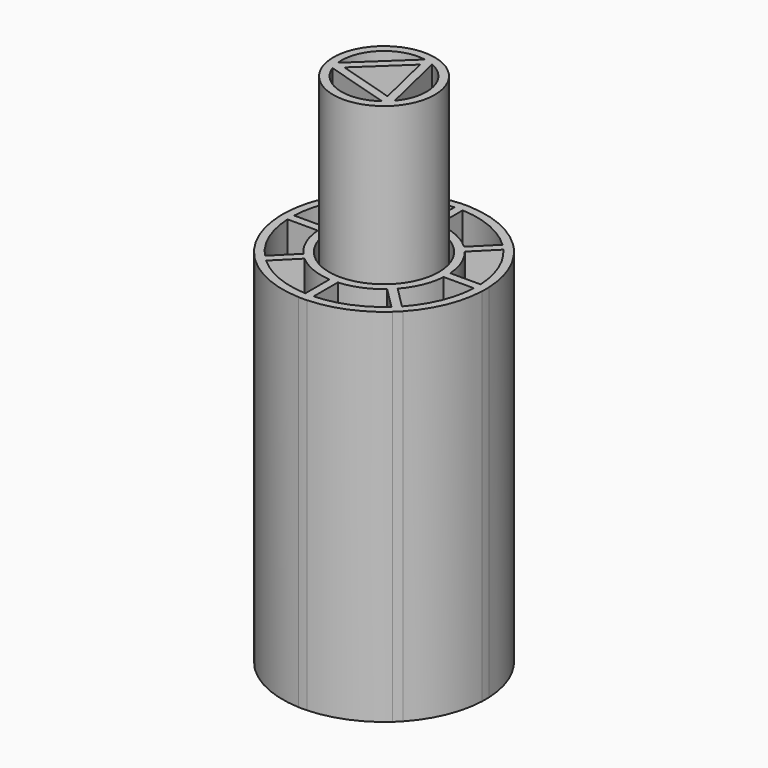
from build123d import *

# Parameters (mm, degrees)
F0_R     = 13.5
F1_DEPTH = 88.9
F0_R_2   = 12.5
F2_DEPTH = 127


# Not quite as in the source:
# - a feature names something its author has since deleted; it is built from what else it names


with BuildPart() as f1:
    # F0 (on Top) → F1 (new body)
    with BuildSketch(Plane.XY):
        with BuildLine():
            ThreePointArc((15.4987343999, -1.016), (15.5236813723, -0.5082722204), (15.532, 0))
            ThreePointArc((15.532, 0), (15.5236813723, 0.5082722204), (15.4987343999, 1.016))
            ThreePointArc((15.4987343999, 1.016), (14.4620963919, 5.664873516), (12.0654338858, 9.7810188195))
            ThreePointArc((12.0654338858, 9.7810188195), (11.3992660397, 10.549870035), (10.6841963244, 11.2734632169))
            ThreePointArc((10.6841963244, 11.2734632169), (6.2198776234, 14.2322221157), (1.016, 15.4987343999))
            ThreePointArc((1.016, 15.4987343999), (0, 15.532), (-1.016, 15.4987343999))
            ThreePointArc((-1.016, 15.4987343999), (-6.2198776234, 14.2322221157), (-10.6841963244, 11.2734632169))
            ThreePointArc((-10.6841963244, 11.2734632169), (-11.3992660397, 10.549870035), (-12.0654338858, 9.7810188195))
            ThreePointArc((-12.0654338858, 9.7810188195), (-14.4620963919, 5.664873516), (-15.4987343999, 1.016))
            ThreePointArc((-15.4987343999, 1.016), (-15.532, 0), (-15.4987343999, -1.016))
            ThreePointArc((-15.4987343999, -1.016), (-14.3311091034, -5.9885170007), (-11.6136432015, -10.3134046555))
            ThreePointArc((-11.6136432015, -10.3134046555), (-10.9141214099, -11.0510170504), (-10.1678472471, -11.7412906599))
            ThreePointArc((-10.1678472471, -11.7412906599), (-5.8990851559, -14.3681529197), (-1.016, -15.4987343999))
            ThreePointArc((-1.016, -15.4987343999), (0, -15.532), (1.016, -15.4987343999))
            ThreePointArc((1.016, -15.4987343999), (5.8990851559, -14.3681529197), (10.1678472471, -11.7412906599))
            ThreePointArc((10.1678472471, -11.7412906599), (10.9141214099, -11.0510170504), (11.6136432015, -10.3134046555))
            ThreePointArc((11.6136432015, -10.3134046555), (14.3311091034, -5.9885170007), (15.4987343999, -1.016))
        make_face()
        Circle(F0_R, mode=Mode.SUBTRACT)
        with BuildLine():
            ThreePointArc((-12.0654338858, 9.7810188195), (-11.3992660397, 10.549870035), (-10.6841963244, 11.2734632169))
            Line((-10.6841963244, 11.2734632169), (-15.9435223337, 16.5327892262))
            ThreePointArc((-15.9435223337, 16.5327892262), (-16.6594901874, 15.8110850575), (-17.3428209151, 15.0584058488))
            Line((-17.3428209151, 15.0584058488), (-12.0654338858, 9.7810188195))
        make_face()
        with BuildLine():
            ThreePointArc((-17.3428209151, 15.0584058488), (-16.6594901874, 15.8110850575), (-15.9435223337, 16.5327892262))
            Line((-15.9435223337, 16.5327892262), (-17.3805805873, 17.9698474798))
            ThreePointArc((-17.3805805873, 17.9698474798), (-18.0967183071, 17.2484430171), (-18.782937732, 16.4985226658))
            Line((-18.782937732, 16.4985226658), (-17.3428209151, 15.0584058488))
        make_face()
        with BuildLine():
            ThreePointArc((-15.4987343999, -1.016), (-15.532, 0), (-15.4987343999, 1.016))
            Line((-15.4987343999, 1.016), (-22.9455173836, 1.016))
            Line((-22.9455173836, 1.016), (-24.9793463485, 1.016))
            ThreePointArc((-24.9793463485, 1.016), (-25, 0), (-24.9793463485, -1.016))
            Line((-24.9793463485, -1.016), (-22.9455173836, -1.016))
            Line((-22.9455173836, -1.016), (-15.4987343999, -1.016))
        make_face()
        with BuildLine():
            ThreePointArc((10.6841963244, 11.2734632169), (11.3992660397, 10.549870035), (12.0654338858, 9.7810188195))
            Line((12.0654338858, 9.7810188195), (17.3428209151, 15.0584058488))
            ThreePointArc((17.3428209151, 15.0584058488), (16.6594901874, 15.8110850575), (15.9435223337, 16.5327892262))
            Line((15.9435223337, 16.5327892262), (10.6841963244, 11.2734632169))
        make_face()
        with BuildLine():
            ThreePointArc((15.9435223337, 16.5327892262), (16.6594901874, 15.8110850575), (17.3428209151, 15.0584058488))
            Line((17.3428209151, 15.0584058488), (18.782937732, 16.4985226658))
            ThreePointArc((18.782937732, 16.4985226658), (18.0967183071, 17.2484430171), (17.3805805873, 17.9698474798))
            Line((17.3805805873, 17.9698474798), (15.9435223337, 16.5327892262))
        make_face()
        with BuildLine():
            ThreePointArc((15.4987343999, 1.016), (15.5236813723, 0.5082722204), (15.532, 0))
            ThreePointArc((15.532, 0), (15.5236813723, -0.5082722204), (15.4987343999, -1.016))
            Line((15.4987343999, -1.016), (22.9455173836, -1.016))
            ThreePointArc((22.9455173836, -1.016), (22.968, 0), (22.9455173836, 1.016))
            Line((22.9455173836, 1.016), (15.4987343999, 1.016))
        make_face()
        with BuildLine():
            Line((24.9793463485, 1.016), (22.9455173836, 1.016))
            ThreePointArc((22.9455173836, 1.016), (22.968, 0), (22.9455173836, -1.016))
            Line((22.9455173836, -1.016), (24.9793463485, -1.016))
            ThreePointArc((24.9793463485, -1.016), (25, 0), (24.9793463485, 1.016))
        make_face()
        with BuildLine():
            ThreePointArc((-1.016, 15.4987343999), (0, 15.532), (1.016, 15.4987343999))
            Line((1.016, 15.4987343999), (1.016, 22.9455173836))
            ThreePointArc((1.016, 22.9455173836), (0, 22.968), (-1.016, 22.9455173836))
            Line((-1.016, 22.9455173836), (-1.016, 15.4987343999))
        make_face()
        with BuildLine():
            ThreePointArc((-1.016, 22.9455173836), (0, 22.968), (1.016, 22.9455173836))
            Line((1.016, 22.9455173836), (1.016, 24.9793463485))
            ThreePointArc((1.016, 24.9793463485), (0, 25), (-1.016, 24.9793463485))
            Line((-1.016, 24.9793463485), (-1.016, 22.9455173836))
        make_face()
        with BuildLine():
            Line((1.016, -24.9793463485), (1.016, -22.9455173836))
            ThreePointArc((1.016, -22.9455173836), (0, -22.968), (-1.016, -22.9455173836))
            Line((-1.016, -22.9455173836), (-1.016, -24.9793463485))
            ThreePointArc((-1.016, -24.9793463485), (0, -25), (1.016, -24.9793463485))
        make_face()
        with BuildLine():
            Line((1.016, -22.9455173836), (1.016, -15.4987343999))
            ThreePointArc((1.016, -15.4987343999), (0, -15.532), (-1.016, -15.4987343999))
            Line((-1.016, -15.4987343999), (-1.016, -22.9455173836))
            ThreePointArc((-1.016, -22.9455173836), (0, -22.968), (1.016, -22.9455173836))
        make_face()
        with BuildLine():
            Line((-15.4350408661, -17.0084842788), (-10.1678472471, -11.7412906599))
            ThreePointArc((-10.1678472471, -11.7412906599), (-10.9141214099, -11.0510170504), (-11.6136432015, -10.3134046555))
            Line((-11.6136432015, -10.3134046555), (-16.8779304911, -15.5776919451))
            ThreePointArc((-16.8779304911, -15.5776919451), (-16.1723165056, -16.309052788), (-15.4350408661, -17.0084842788))
        make_face()
        with BuildLine():
            Line((-16.8734331332, -18.4468765459), (-15.4350408661, -17.0084842788))
            ThreePointArc((-15.4350408661, -17.0084842788), (-16.1723165056, -16.309052788), (-16.8779304911, -15.5776919451))
            Line((-16.8779304911, -15.5776919451), (-18.3158302672, -17.0155917212))
            ThreePointArc((-18.3158302672, -17.0155917212), (-17.6091796722, -17.7458950542), (-16.8734331332, -18.4468765459))
        make_face()
        with BuildLine():
            Line((16.8779304911, -15.5776919451), (11.6136432015, -10.3134046555))
            ThreePointArc((11.6136432015, -10.3134046555), (10.9141214099, -11.0510170504), (10.1678472471, -11.7412906599))
            Line((10.1678472471, -11.7412906599), (15.4350408661, -17.0084842788))
            ThreePointArc((15.4350408661, -17.0084842788), (16.1723165056, -16.309052788), (16.8779304911, -15.5776919451))
        make_face()
        with BuildLine():
            Line((18.3158302672, -17.0155917212), (16.8779304911, -15.5776919451))
            ThreePointArc((16.8779304911, -15.5776919451), (16.1723165056, -16.309052788), (15.4350408661, -17.0084842788))
            Line((15.4350408661, -17.0084842788), (16.8734331332, -18.4468765459))
            ThreePointArc((16.8734331332, -18.4468765459), (17.6091796722, -17.7458950542), (18.3158302672, -17.0155917212))
        make_face()
        with BuildLine():
            Line((16.8734331332, -18.4468765459), (15.4350408661, -17.0084842788))
            ThreePointArc((15.4350408661, -17.0084842788), (8.7447856987, -21.2381201401), (1.016, -22.9455173836))
            Line((1.016, -22.9455173836), (1.016, -24.9793463485))
            ThreePointArc((1.016, -24.9793463485), (9.5224075153, -23.1154440821), (16.8734331332, -18.4468765459))
        make_face()
        with BuildLine():
            Line((24.9793463485, -1.016), (22.9455173836, -1.016))
            ThreePointArc((22.9455173836, -1.016), (21.2011195042, -8.8341131851), (16.8779304911, -15.5776919451))
            Line((16.8779304911, -15.5776919451), (18.3158302672, -17.0155917212))
            ThreePointArc((18.3158302672, -17.0155917212), (23.0784491108, -9.6117213152), (24.9793463485, -1.016))
        make_face()
        with BuildLine():
            ThreePointArc((17.3428209151, 15.0584058488), (21.3327176239, 8.5114148517), (22.9455173836, 1.016))
            Line((22.9455173836, 1.016), (24.9793463485, 1.016))
            ThreePointArc((24.9793463485, 1.016), (23.2101594999, 9.2891601336), (18.782937732, 16.4985226658))
            Line((18.782937732, 16.4985226658), (17.3428209151, 15.0584058488))
        make_face()
        with BuildLine():
            Line((-1.016, -24.9793463485), (-1.016, -22.9455173836))
            ThreePointArc((-1.016, -22.9455173836), (-8.7447856987, -21.2381201401), (-15.4350408661, -17.0084842788))
            Line((-15.4350408661, -17.0084842788), (-16.8734331332, -18.4468765459))
            ThreePointArc((-16.8734331332, -18.4468765459), (-9.5224075153, -23.1154440821), (-1.016, -24.9793463485))
        make_face()
        with BuildLine():
            Line((-18.3158302672, -17.0155917212), (-16.8779304911, -15.5776919451))
            ThreePointArc((-16.8779304911, -15.5776919451), (-21.2011195042, -8.8341131851), (-22.9455173836, -1.016))
            Line((-22.9455173836, -1.016), (-24.9793463485, -1.016))
            ThreePointArc((-24.9793463485, -1.016), (-23.0784491108, -9.6117213152), (-18.3158302672, -17.0155917212))
        make_face()
        with BuildLine():
            ThreePointArc((-22.9455173836, 1.016), (-21.3327176239, 8.5114148517), (-17.3428209151, 15.0584058488))
            Line((-17.3428209151, 15.0584058488), (-18.782937732, 16.4985226658))
            ThreePointArc((-18.782937732, 16.4985226658), (-23.2101594999, 9.2891601336), (-24.9793463485, 1.016))
            Line((-24.9793463485, 1.016), (-22.9455173836, 1.016))
        make_face()
        with BuildLine():
            ThreePointArc((-15.9435223337, 16.5327892262), (-9.065711227, 21.1031254545), (-1.016, 22.9455173836))
            Line((-1.016, 22.9455173836), (-1.016, 24.9793463485))
            ThreePointArc((-1.016, 24.9793463485), (-9.8433639029, 22.9806045846), (-17.3805805873, 17.9698474798))
            Line((-17.3805805873, 17.9698474798), (-15.9435223337, 16.5327892262))
        make_face()
        with BuildLine():
            ThreePointArc((1.016, 22.9455173836), (9.065711227, 21.1031254545), (15.9435223337, 16.5327892262))
            Line((15.9435223337, 16.5327892262), (17.3805805873, 17.9698474798))
            ThreePointArc((17.3805805873, 17.9698474798), (9.8433639029, 22.9806045846), (1.016, 24.9793463485))
            Line((1.016, 24.9793463485), (1.016, 22.9455173836))
        make_face()
    extrude(amount=F1_DEPTH)


with BuildPart() as f2:
    # F0 (on Top) → F2 (new body)
    with BuildSketch(Plane.XY):
        Circle(F0_R_2)
        with BuildLine():
            ThreePointArc((4.1556189742, 9.6078017747), (8.748715432, 5.7479563576), (10.468, 0))
            ThreePointArc((10.468, 0), (9.8344886963, -3.5863429958), (8.010633534, -6.7386032963))
            ThreePointArc((8.010633534, -6.7386032963), (7.1751231328, -7.6221146691), (6.2427909243, -8.4027724874))
            ThreePointArc((6.2427909243, -8.4027724874), (-3.0133833676, -10.0248962428), (-9.8411184076, -3.5681104927))
            ThreePointArc((-9.8411184076, -3.5681104927), (-10.1885065004, -2.4027815737), (-10.3984098985, -1.2050292872))
            ThreePointArc((-10.3984098985, -1.2050292872), (-7.1751231328, 7.6221146691), (1.8304848736, 10.306713789))
            ThreePointArc((1.8304848736, 10.306713789), (3.0133833676, 10.0248962428), (4.1556189742, 9.6078017747))
        make_face(mode=Mode.SUBTRACT)
        with BuildLine():
            Line((8.010633534, -6.7386032963), (4.1556189742, 9.6078017747))
            ThreePointArc((4.1556189742, 9.6078017747), (3.0133833676, 10.0248962428), (1.8304848736, 10.306713789))
            Line((1.8304848736, 10.306713789), (-10.3984098985, -1.2050292872))
            ThreePointArc((-10.3984098985, -1.2050292872), (-10.1885065004, -2.4027815737), (-9.8411184076, -3.5681104927))
            Line((-9.8411184076, -3.5681104927), (6.2427909243, -8.4027724874))
            ThreePointArc((6.2427909243, -8.4027724874), (7.1751231328, -7.6221146691), (8.010633534, -6.7386032963))
        make_face()
        Polygon((5.7823212408, -6.1425448365), (-8.2107604927, -1.9363646691), (2.4284392519, 8.0789095056), align=None, mode=Mode.SUBTRACT)
    extrude(amount=F2_DEPTH)


solid = Compound([f1.part, f2.part])
